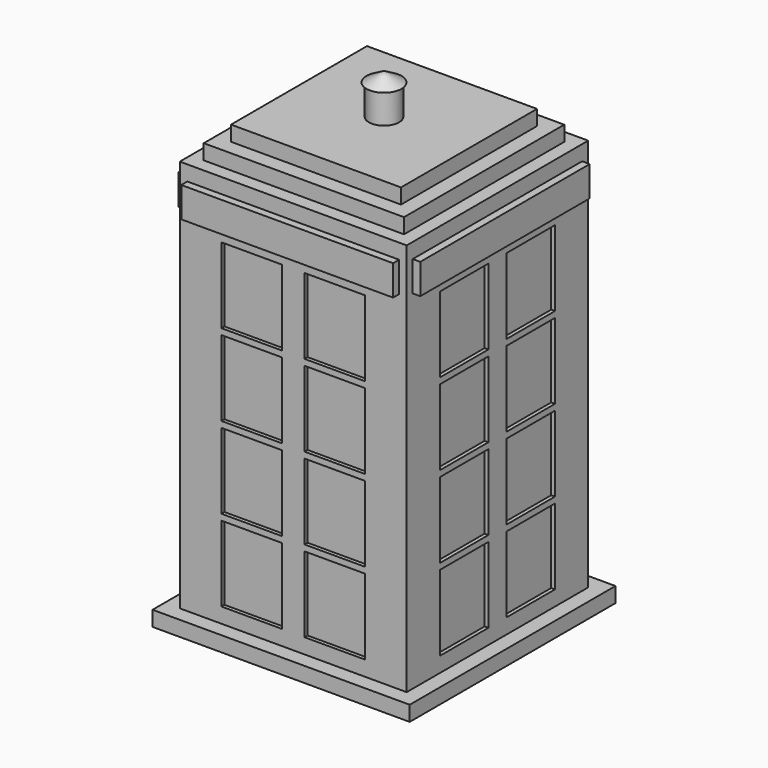
from build123d import *

# Parameters (mm, degrees)
F0_W             = 107.95
F0_H             = 107.95
F1_DEPTH         = 6.35
F2_W             = 95.25
F2_H             = 95.25
F3_DEPTH         = 165.1
F4_W             = 84.073998034
F4_H             = 84.073998034
F5_DEPTH         = 6.35
F6_W             = 71.373998034
F6_H             = 71.373998034
F7_DEPTH         = 6.35
F8_W             = 88.9
F8_H             = 12.7
F9_DEPTH         = 3.175
F9_COPIES_COUNT  = 4
F11_R            = 6.35
F12_DEPTH        = 12.7
F13_R            = 7.366000209
F14_DEPTH        = 25.4
F14_TAPER        = 60
F15_W            = 25.4
F15_H            = 31.75
F16_DEPTH        = 1.5875
F16_COPIES_COUNT = 4


# Not quite as in the source:
# - a pattern or mirror of a feature is missing from the dataset's text; its kind, count and spacing are read off the source's solid


with BuildPart() as f1:
    # F0 (on Top) → F1 (new body)
    with BuildSketch(Plane.XY):
        Rectangle(F0_W, F0_H)
    extrude(amount=F1_DEPTH)

    # F2 (on face) → F3 (join)
    with BuildSketch(Plane.XY.offset(6.35)):
        Rectangle(F2_W, F2_H)
    extrude(amount=F3_DEPTH)

    # F4 (on face) → F5 (join)
    with BuildSketch(Plane.XY.offset(171.45)):
        Rectangle(F4_W, F4_H)
    extrude(amount=F5_DEPTH)

    # F6 (on face) → F7 (join)
    with BuildSketch(Plane.XY.offset(177.8)):
        Rectangle(F6_W, F6_H)
    extrude(amount=F7_DEPTH)

    # F8 (on face) → F9 (join)
    with BuildSketch(Plane(origin=(-47.625, 0, 0), x_dir=(0, -1, 0), z_dir=(-1, 0, 0))):
        with Locations((0, 158.7718427181)):
            Rectangle(F8_W, F8_H)
    f9 = extrude(amount=F9_DEPTH)

    # F9_copies: F9 ×4 about axis
    f9_copies_axis = Axis((0, 0, 0), (0, 0, 1))
    for i in range(1, F9_COPIES_COUNT):
        add(f9.rotate(f9_copies_axis, i * 360 / F9_COPIES_COUNT))

    # F11 (on face) → F12 (join)
    with BuildSketch(Plane.XY.offset(184.15)):
        Circle(F11_R)
    extrude(amount=F12_DEPTH)

    # F13 (on face) → F14 (join)
    with BuildSketch(Plane.XY.offset(196.85)):
        Circle(F13_R)
    extrude(amount=F14_DEPTH, taper=F14_TAPER)

    # F15 (on face) → F16 (cut)
    with BuildSketch(Plane.XZ.offset(47.625)):
        with Locations((-17.4625, 28.575)):
            Rectangle(F15_W, F15_H)
        with Locations((-17.4625, 62.865)):
            Rectangle(F15_W, F15_H)
        with Locations((-17.4625, 97.155)):
            Rectangle(F15_W, F15_H)
        with Locations((-17.4625, 131.445)):
            Rectangle(F15_W, F15_H)
        with Locations((17.4625, 97.155)):
            Rectangle(F15_W, F15_H)
        with Locations((17.4625, 131.445)):
            Rectangle(F15_W, F15_H)
        with Locations((17.4625, 62.865)):
            Rectangle(F15_W, F15_H)
        with Locations((17.4625, 28.575)):
            Rectangle(F15_W, F15_H)
    f16 = extrude(amount=-F16_DEPTH, mode=Mode.SUBTRACT)

    # F16_copies: F16 ×4 about axis
    f16_copies_axis = Axis((0, 0, 0), (0, 0, 1))
    for i in range(1, F16_COPIES_COUNT):
        add(f16.rotate(f16_copies_axis, i * 360 / F16_COPIES_COUNT), mode=Mode.SUBTRACT)


solid = f1.part
